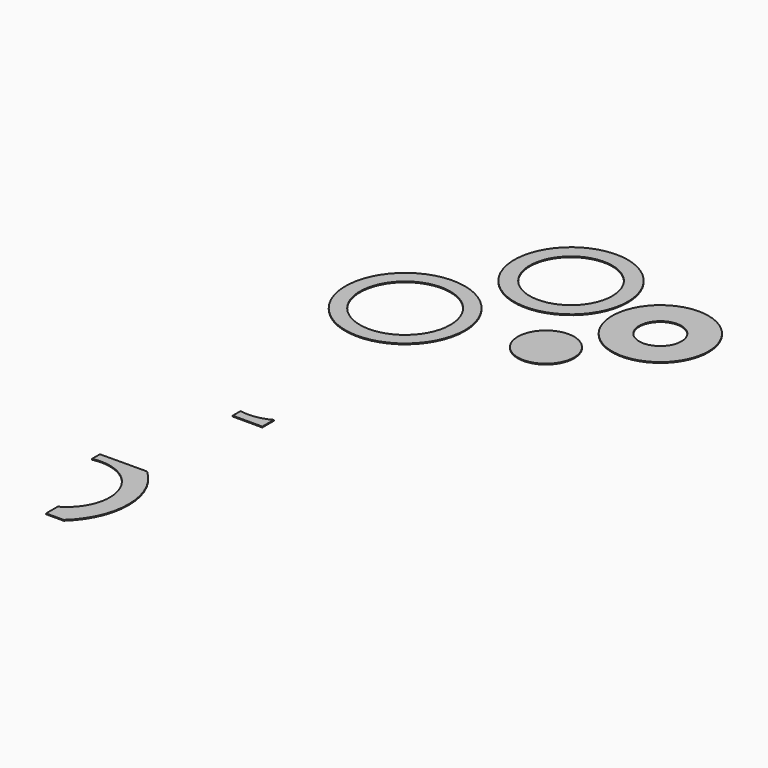
from build123d import *

# Parameters (mm, degrees)
F0_R      = 600
F1_DEPTH  = 18
F2_R      = 1027
F2_R_2    = 450
F3_DEPTH  = 18
F4_R      = 1210
F4_R_2    = 880
F5_DEPTH  = 18
F6_R      = 1272.5
F6_R_2    = 965
F7_DEPTH  = 18
F9_DEPTH  = 18
F11_DEPTH = 18


with BuildPart() as f1:
    # F0 (on Top) → F1 (new body)
    with BuildSketch(Plane.XY):
        Circle(F0_R)
    extrude(amount=F1_DEPTH)


with BuildPart() as f3:
    # F2 (on Top) → F3 (new body)
    with BuildSketch(Plane.XY):
        with Locations((1183.201789856, 1567.84760952)):
            Circle(F2_R)
        with Locations((1183.201789856, 1567.84760952)):
            Circle(F2_R_2, mode=Mode.SUBTRACT)
    extrude(amount=F3_DEPTH)


with BuildPart() as f5:
    # F4 (on Top) → F5 (new body)
    with BuildSketch(Plane.XY):
        with Locations((-1167.2713756561, 2126.6794204712)):
            Circle(F4_R)
        with Locations((-1167.2713756561, 2126.6794204712)):
            Circle(F4_R_2, mode=Mode.SUBTRACT)
    extrude(amount=F5_DEPTH)


with BuildPart() as f7:
    # F6 (on Top) → F7 (new body)
    with BuildSketch(Plane.XY):
        with Locations((-2705.9388160706, -369.3017959595)):
            Circle(F6_R)
        with Locations((-2705.9388160706, -369.3017959595)):
            Circle(F6_R_2, mode=Mode.SUBTRACT)
    extrude(amount=F7_DEPTH)


with BuildPart() as f9:
    # F8 (on Top) → F9 (new body)
    with BuildSketch(Plane.XY):
        with BuildLine():
            ThreePointArc((-1896.1358144379, -4877.4950429265), (-2202.9667353597, -4983.8530885251), (-2527.6358144379, -4976.9801715458))
            Line((-2527.6358144379, -4976.9801715458), (-2527.6358144379, -5187.0612450341))
            Line((-2527.6358144379, -5187.0612450341), (-1896.1358144379, -5187.0612450341))
            Line((-1896.1358144379, -5187.0612450341), (-1896.1358144379, -4877.4950429265))
        make_face()
    extrude(amount=F9_DEPTH)


with BuildPart() as f11:
    # F10 (on face) → F11 (new body)
    with BuildSketch(Plane.XY):
        with BuildLine():
            ThreePointArc((-3383.762090595, -7864.2263730014), (-2339.5758122783, -8446.5011454854), (-2752.262090595, -9568.5790974055))
            Line((-2752.262090595, -9568.5790974055), (-2752.262090595, -9878.1452995131))
            Line((-2752.262090595, -9878.1452995131), (-2498.4145172777, -9878.1452995131))
            Line((-2498.4145172777, -9878.1452995131), (-2377.0565725809, -9878.1452995131))
            ThreePointArc((-2377.0565725809, -9878.1452995131), (-1883.7679503047, -8761.952556401), (-2383.2887193923, -7648.5348872878))
            Line((-2383.2887193923, -7648.5348872878), (-3383.762090595, -7654.1452995131))
            Line((-3383.762090595, -7654.1452995131), (-3383.762090595, -7864.2263730014))
        make_face()
    extrude(amount=F11_DEPTH)


solid = Compound([f1.part, f3.part, f5.part, f7.part, f9.part, f11.part])
